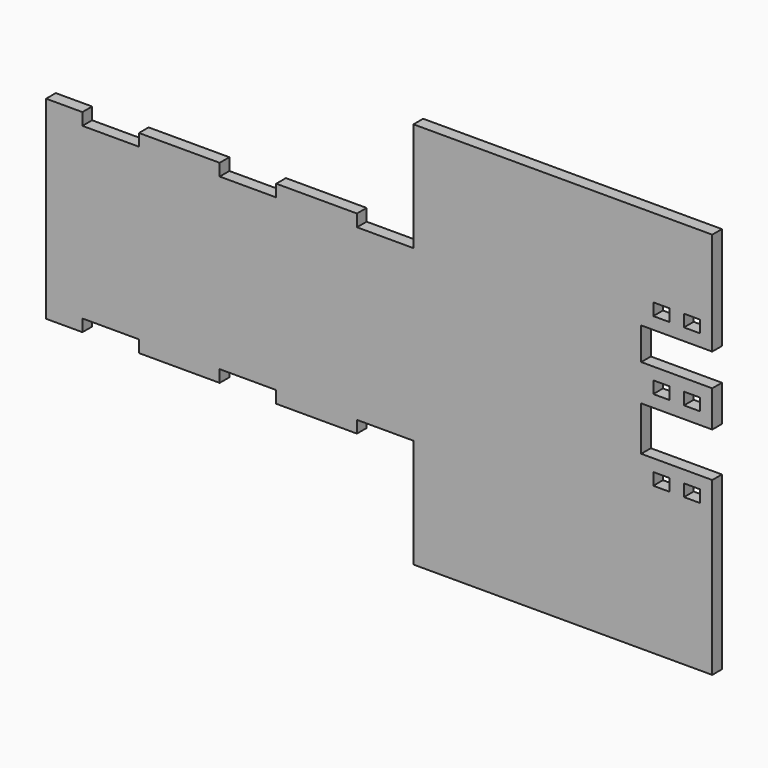
from build123d import *

# Parameters (mm, degrees)
F0_W     = 25.4
F0_H     = 19.05
F0_W_2   = 469.9
F0_H_2   = 152.4
F0_W_3   = 111.76
F0_H_3   = 57.15
F1_DEPTH = 19.05


# Not quite as in the source:
# - a feature names something its author has since deleted; it is built from what else it names


with BuildPart() as f1:
    # F0 (on Front) → F1 (new body)
    with BuildSketch(Plane.XZ):
        Polygon((-448.4900477648, 138.0508303034), (-505.6400477648, 138.0508303034), (-505.6400477648, -166.7491696966), (-448.4900477648, -166.7491696966), (-448.4900477648, -147.6991696966), (-359.5900477648, -147.6991696966), (-359.5900477648, -166.7491696966), (-232.5900477648, -166.7491696966), (-232.5900477648, -147.6991696966), (-143.6900477648, -147.6991696966), (-143.6900477648, -166.7491696966), (-16.6900477648, -166.7491696966), (-16.6900477648, -147.6991696966), (72.2099522352, -147.6991696966), (72.2099522352, -166.7491696966), (542.1099522352, -166.7491696966), (542.1099522352, -49.2741696966), (523.0599522352, -49.2741696966), (497.6599522352, -49.2741696966), (474.7999522352, -49.2741696966), (449.3999522352, -49.2741696966), (430.3499522352, -49.2741696966), (430.3499522352, -23.8741696966), (430.3499522352, 20.5758303034), (430.3499522352, 77.7258303034), (430.3499522352, 90.4258303034), (430.3499522352, 128.5258303034), (449.3999522352, 128.5258303034), (474.7999522352, 128.5258303034), (497.6599522352, 128.5258303034), (523.0599522352, 128.5258303034), (542.1099522352, 128.5258303034), (542.1099522352, 138.0508303034), (474.7999522352, 138.0508303034), (449.3999522352, 138.0508303034), (72.2099522352, 138.0508303034), (72.2099522352, 119.0008303034), (-16.6900477648, 119.0008303034), (-16.6900477648, 138.0508303034), (-143.6900477648, 138.0508303034), (-143.6900477648, 119.0008303034), (-232.5900477648, 119.0008303034), (-232.5900477648, 138.0508303034), (-359.5900477648, 138.0508303034), (-359.5900477648, 119.0008303034), (-448.4900477648, 119.0008303034), align=None)
        with Locations((462.0999522352, -77.8491696966)):
            Rectangle(F0_W, F0_H, mode=Mode.SUBTRACT)
        with Locations((510.3599522352, -77.8491696966)):
            Rectangle(F0_W, F0_H, mode=Mode.SUBTRACT)
        with Locations((307.1599522352, -242.9491696966)):
            Rectangle(F0_W_2, F0_H_2)
        Polygon((72.2099522352, 290.4508303034), (72.2099522352, 138.0508303034), (449.3999522352, 138.0508303034), (474.7999522352, 138.0508303034), (542.1099522352, 138.0508303034), (542.1099522352, 290.4508303034), align=None)
        with Locations((462.0999522352, 157.1008303034)):
            Rectangle(F0_W, F0_H, mode=Mode.SUBTRACT)
        with Locations((510.3599522352, 157.1008303034)):
            Rectangle(F0_W, F0_H, mode=Mode.SUBTRACT)
        with Locations((486.2299522352, 49.1508303034)):
            Rectangle(F0_W_3, F0_H_3)
        with Locations((462.0999522352, 49.1508303034)):
            Rectangle(F0_W, F0_H, mode=Mode.SUBTRACT)
        with Locations((510.3599522352, 49.1508303034)):
            Rectangle(F0_W, F0_H, mode=Mode.SUBTRACT)
    extrude(amount=F1_DEPTH)


solid = f1.part
